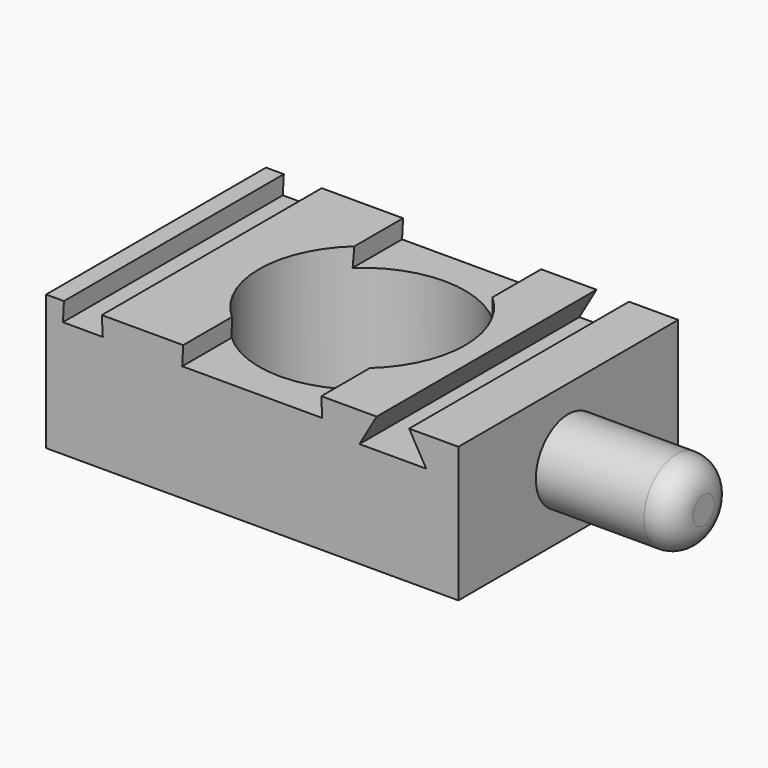
from build123d import *

# Parameters (mm, degrees)
F0_W                     = 76.2
F0_H                     = 50.8
F0_R                     = 19.05
F1_DEPTH                 = 25
F2_W                     = 7
F2_H                     = 50.8
F3_DEPTH                 = 3.5
DRAFT_F3_DRAFTED_ANGLE   = -3
DRAFT_F3_2_DRAFTED_ANGLE = -3
DRAFT_F3_3_DRAFTED_ANGLE = -3
F5_DEPTH                 = 50.801
F6_R                     = 7.5
F7_DEPTH                 = 25
F8_R                     = 5


# Not quite as in the source:
# - an extrude with a draft is written as a straight extrude whose walls are then drafted


with BuildPart() as f1:
    # F0 (on Top) → F1 (new body)
    with BuildSketch(Plane.XY):
        Rectangle(F0_W, F0_H)
        Circle(F0_R, mode=Mode.SUBTRACT)
    extrude(amount=F1_DEPTH)


with BuildPart() as f3_drafted:
    # F2 (on face) → F3 (new body)
    with BuildSketch(Plane.XY.offset(25)):
        with Locations((-31.3, 0)):
            Rectangle(F2_W, F2_H)
    extrude(amount=-F3_DEPTH)

    # draft_F3_drafted
    draft_f3_drafted_walls = [f3_drafted.faces().sort_by_distance(p)[0] for p in [
        (-31.3, 25.4, 22.6666666667),
        (-34.8, 0, 22.6666666667),
        (-31.3, -25.4, 22.6666666667),
        (-27.8, 0, 22.6666666667),
    ]]
    draft(draft_f3_drafted_walls, neutral_plane=Plane(origin=(0, 0, 25), x_dir=(1, 0, 0), z_dir=(0, 0, -1)), angle=DRAFT_F3_DRAFTED_ANGLE)


with BuildPart() as f1_1:
    add(f1.part)

    # join_F3_drafted: cut F3_drafted
    add(f3_drafted.part, mode=Mode.SUBTRACT)


with BuildPart() as f3_2_drafted:
    # F2 (on face) → F3, piece 2 (new body)
    with BuildSketch(Plane.XY.offset(25)):
        with BuildLine():
            Line((-12.7599649131, -14.1451686245), (-12.7599649131, -25.4))
            Line((-12.7599649131, -25.4), (12.7599649131, -25.4))
            Line((12.7599649131, -25.4), (12.7599649131, -14.1451686245))
            ThreePointArc((12.7599649131, -14.1451686245), (0, -19.05), (-12.7599649131, -14.1451686245))
        make_face()
    extrude(amount=-F3_DEPTH)

    # draft_F3_2_drafted
    draft_f3_2_drafted_walls = [f3_2_drafted.faces().sort_by_distance(p)[0] for p in [
        (-12.7599649131, -19.7725843123, 22.6666666667),
        (0, -25.4, 22.6666666667),
        (12.7599649131, -19.7725843123, 22.6666666667),
        (0, -19.05, 22.6666666667),
    ]]
    draft(draft_f3_2_drafted_walls, neutral_plane=Plane(origin=(0, 0, 25), x_dir=(1, 0, 0), z_dir=(0, 0, -1)), angle=DRAFT_F3_2_DRAFTED_ANGLE)


with BuildPart() as f1_2:
    add(f1_1.part)

    # join_F3_2_drafted: cut F3_2_drafted
    add(f3_2_drafted.part, mode=Mode.SUBTRACT)


with BuildPart() as f3_3_drafted:
    # F2 (on face) → F3, piece 3 (new body)
    with BuildSketch(Plane.XY.offset(25)):
        with BuildLine():
            Line((12.7599649131, 25.4), (-12.7599649131, 25.4))
            Line((-12.7599649131, 25.4), (-12.7599649131, 14.1451686245))
            ThreePointArc((-12.7599649131, 14.1451686245), (0, 19.05), (12.7599649131, 14.1451686245))
            Line((12.7599649131, 14.1451686245), (12.7599649131, 25.4))
        make_face()
    extrude(amount=-F3_DEPTH)

    # draft_F3_3_drafted
    draft_f3_3_drafted_walls = [f3_3_drafted.faces().sort_by_distance(p)[0] for p in [
        (0, 19.05, 22.6666666667),
        (12.7599649131, 19.7725843123, 22.6666666667),
        (0, 25.4, 22.6666666667),
        (-12.7599649131, 19.7725843123, 22.6666666667),
    ]]
    draft(draft_f3_3_drafted_walls, neutral_plane=Plane(origin=(0, 0, 25), x_dir=(1, 0, 0), z_dir=(0, 0, -1)), angle=DRAFT_F3_3_DRAFTED_ANGLE)


with BuildPart() as f1_3:
    add(f1_2.part)

    # join_F3_3_drafted: cut F3_3_drafted
    add(f3_3_drafted.part, mode=Mode.SUBTRACT)

    # F4 (on face) → F5 (cut, through all)
    with BuildSketch(Plane.XZ.offset(25.4)):
        Polygon((29, 25), (23, 25), (19.8245735195, 19.5), (32.1754264805, 19.5), align=None)
    extrude(amount=-F5_DEPTH, mode=Mode.SUBTRACT)

    # F6 (on face) → F7 (join)
    with BuildSketch(Plane.YZ.offset(38.1)):
        with Locations((0, 12.5)):
            Circle(F6_R)
    extrude(amount=F7_DEPTH)

    # F8
    f8_edges = [f1_3.edges().sort_by_distance(p)[0] for p in [
        (63.1, -7.5, 12.5),
    ]]
    fillet(f8_edges, radius=F8_R)


solid = f1_3.part
